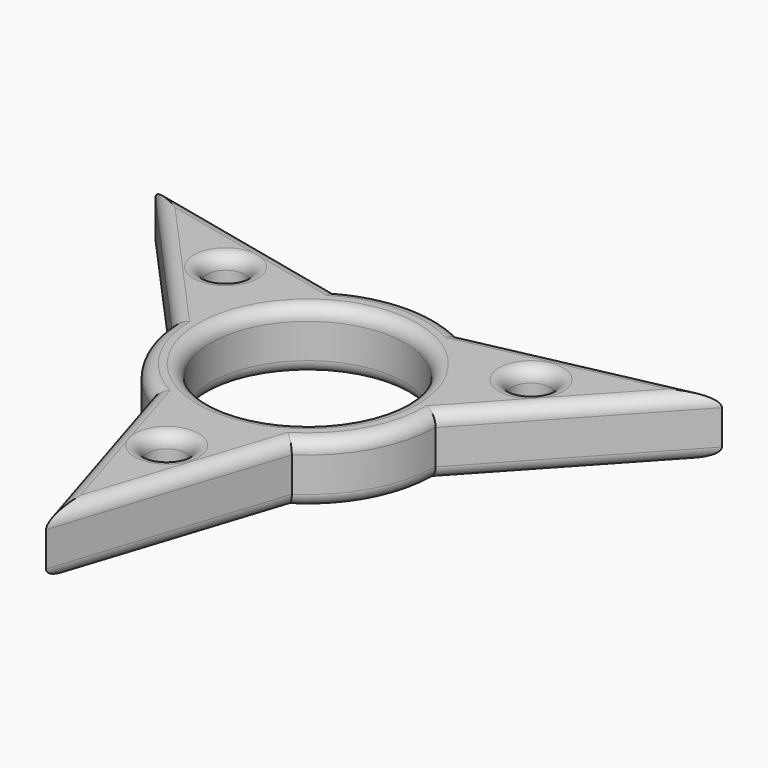
from build123d import *

# Parameters (mm, degrees)
F0_R          = 2.2
F0_R_2        = 11.2
F1_DEPTH      = 7
F2_T4_DEPTH   = 34.0623272755
F2_S5_R       = 15
F2_T6_DEPTH   = 19
F2_T10_ANGLE  = 84.4962693164
F2_T16_DEPTH  = 33.6377133372
F2_S17_R      = 15
F2_T18_DEPTH  = 19
F2_T22_DEPTH  = 34.0623272755
F2_S23_R      = 15
F2_T24_DEPTH  = 19
F2_T28_ANGLE  = 84.4962693164
F2_T34_DEPTH  = 33.6377133372
F2_S35_R      = 15
F2_T36_DEPTH  = 19
F2_T40_DEPTH  = 34.0623272755
F2_S41_R      = 15
F2_T42_DEPTH  = 19
F2_T46_ANGLE  = 84.4962693164
F2_T52_DEPTH  = 33.6377133372
F2_S53_R      = 15
F2_T54_DEPTH  = 19
F2_T66_DEPTH  = 34.0623272755
F2_S67_R      = 15
F2_T68_DEPTH  = 19
F2_T72_ANGLE  = 84.4962693164
F2_T78_DEPTH  = 33.6377133372
F2_S79_R      = 15
F2_T80_DEPTH  = 19
F2_T84_DEPTH  = 34.0623272755
F2_S85_R      = 15
F2_T86_DEPTH  = 19
F2_T90_ANGLE  = 84.4962693164
F2_T96_DEPTH  = 33.6377133372
F2_S97_R      = 15
F2_T98_DEPTH  = 19
F2_T102_DEPTH = 34.0623272755
F2_S103_R     = 15
F2_T104_DEPTH = 19
F2_T108_ANGLE = 84.4962693164
F2_T114_DEPTH = 33.6377133372
F2_S115_R     = 15
F2_T116_DEPTH = 19
F2_T129_DEPTH = 34.0623272755
F2_S130_R     = 15
F2_T131_DEPTH = 19
F2_T134_ANGLE = 84.4962693164
F2_T142_ANGLE = 84.4962693164
F2_T147_DEPTH = 33.6377133372
F2_S148_R     = 15
F2_T149_DEPTH = 19
F2_T155_DEPTH = 34.0623272755
F2_S156_R     = 15
F2_T157_DEPTH = 19
F2_T160_ANGLE = 84.4962693164
F2_T168_ANGLE = 84.4962693164
F2_T173_DEPTH = 33.6377133372
F2_S174_R     = 15
F2_T175_DEPTH = 19
F2_T181_DEPTH = 34.0623272755
F2_S182_R     = 15
F2_T183_DEPTH = 19
F2_T186_ANGLE = 84.4962693164
F2_T194_ANGLE = 84.4962693164
F2_T199_DEPTH = 33.6377133372
F2_S200_R     = 15
F2_T201_DEPTH = 19
F2_T207_DEPTH = 34.0623272755
F2_S208_R     = 15
F2_T209_DEPTH = 19
F2_T212_ANGLE = 84.4962693164
F2_T220_ANGLE = 84.4962693164
F2_T225_DEPTH = 33.6377133372
F2_S226_R     = 15
F2_T227_DEPTH = 19
F2_T233_DEPTH = 34.0623272755
F2_S234_R     = 15
F2_T235_DEPTH = 19
F2_T238_ANGLE = 84.4962693164
F2_T246_ANGLE = 84.4962693164
F2_T251_DEPTH = 33.6377133372
F2_S252_R     = 15
F2_T253_DEPTH = 19
F2_T259_DEPTH = 34.0623272755
F2_S260_R     = 15
F2_T261_DEPTH = 19
F2_T264_ANGLE = 84.4962693164
F2_T272_ANGLE = 84.4962693164
F2_T277_DEPTH = 33.6377133372
F2_S278_R     = 15
F2_T279_DEPTH = 19


# Not quite as in the source:
# - a fillet or chamfer that OpenCascade refuses, or shapes differently, is made with other operations: its cross-section is extruded or revolved along the edge and cut away or added


with BuildPart() as f1:
    # F0 (on Top) → F1 (new body)
    with BuildSketch(Plane.XY):
        with BuildLine():
            Line((-32.7569814166, 18.9122520387), (-14.9774534352, -0.8221244411))
            ThreePointArc((-14.9774534352, -0.8221244411), (-12.8488944768, -7.7398908729), (-7.7287556481, -12.8555955184))
            Line((-7.7287556481, -12.8555955184), (0, -37.8245040774))
            Line((0, -37.8245040774), (8.2007073687, -12.5597929383))
            ThreePointArc((8.2007073687, -12.5597929383), (13.1273893569, -7.2575235909), (14.9976501237, -0.2655009717))
            Line((14.9976501237, -0.2655009717), (32.7569814166, 18.9122520387))
            Line((32.7569814166, 18.9122520387), (6.7767460665, 13.3819173794))
            ThreePointArc((6.7767460665, 13.3819173794), (-0.2784948801, 14.9974144639), (-7.2688944757, 13.1210964901))
            Line((-7.2688944757, 13.1210964901), (-32.7569814166, 18.9122520387))
        make_face()
        with Locations((0, -20.3903708607)):
            Circle(F0_R, mode=Mode.SUBTRACT)
        Circle(F0_R_2, mode=Mode.SUBTRACT)
        with Locations((-17.6585791579, 10.1951854303)):
            Circle(F0_R, mode=Mode.SUBTRACT)
        with Locations((17.6585791579, 10.1951854303)):
            Circle(F0_R, mode=Mode.SUBTRACT)
    extrude(amount=F1_DEPTH)

    # F2: fillet of radius 1.5 on 26 edges, made by hand


with BuildPart() as f2_tool2:
    # F2_s3 → F2_t4 (new body)
    with BuildSketch(Plane(origin=(-26.5911251268, 29.5148034764, 0), x_dir=(0, 0, 1), z_dir=(0.6693512883, -0.7429460632, 0))):
        with BuildLine():
            ThreePointArc((5.5, 11.6777301208), (6.5606601718, 11.2383902926), (7, 10.1777301208))
            Line((7, 10.1777301208), (7, 11.6777301208))
            Line((7, 11.6777301208), (5.5, 11.6777301208))
        make_face()
    extrude(amount=F2_T4_DEPTH)

    # F2_s5 → F2_t6 (cut, symmetric)
    with BuildSketch(Plane.XY.offset(6.2)):
        Circle(F2_S5_R)
    extrude(amount=F2_T6_DEPTH, both=True, mode=Mode.SUBTRACT)


with BuildPart() as f1_1:
    add(f1.part)

    # F2_t1: cut F2_tool2
    add(f2_tool2.part, mode=Mode.SUBTRACT)


with BuildPart() as f2_tool8:
    # F2_s9 → F2_t10 (revolve)
    with BuildSketch(Plane(origin=(0, 0, 0), x_dir=(0, 0, 1), z_dir=(0.1939655707, 0.9810083371, 0))):
        with BuildLine():
            ThreePointArc((5.5, -15), (6.5606601718, -14.5606601718), (7, -13.5))
            Line((7, -13.5), (7, -15))
            Line((7, -15), (5.5, -15))
        make_face()
    revolve(axis=Axis((0, 0, 7), (0, 0, 1)), revolution_arc=F2_T10_ANGLE)

    split(bisect_by=Plane(origin=(-8.6759236209, -7.8165037005, 0), x_dir=(0, 0, 1), z_dir=(-0.7429460632, -0.6693512883, 0)), keep=Keep.TOP)

    split(bisect_by=Plane(origin=(-10.6843276365, -3.3071752965, 0), x_dir=(0, 0, 1), z_dir=(-0.9552828221, -0.2956936419, 0)), keep=Keep.TOP)


with BuildPart() as f1_2:
    add(f1_1.part)

    # F2_t7: cut F2_tool8
    add(f2_tool8.part, mode=Mode.SUBTRACT)


with BuildPart() as f2_tool14:
    # F2_s15 → F2_t16 (new body)
    with BuildSketch(Plane(origin=(1.8467208313, -5.9661096392, 0), x_dir=(0, 0, 1), z_dir=(0.2956936419, -0.9552828221, 0))):
        with BuildLine():
            ThreePointArc((5.5, 11.1844653644), (6.5606601718, 10.7451255361), (7, 9.6844653644))
            Line((7, 9.6844653644), (7, 11.1844653644))
            Line((7, 11.1844653644), (5.5, 11.1844653644))
        make_face()
    extrude(amount=F2_T16_DEPTH)

    # F2_s17 → F2_t18 (cut, symmetric)
    with BuildSketch(Plane.XY.offset(6.2)):
        Circle(F2_S17_R)
    extrude(amount=F2_T18_DEPTH, both=True, mode=Mode.SUBTRACT)


with BuildPart() as f1_3:
    add(f1_2.part)

    # F2_t13: cut F2_tool14
    add(f2_tool14.part, mode=Mode.SUBTRACT)


with BuildPart() as f2_tool20:
    # F2_s21 → F2_t22 (new body)
    with BuildSketch(Plane(origin=(-12.2650070349, -37.7859916132, 0), x_dir=(0, 0, 1), z_dir=(0.3087345203, 0.9511482513, 0))):
        with BuildLine():
            ThreePointArc((5.5, 11.6777301208), (6.5606601718, 11.2383902926), (7, 10.1777301208))
            Line((7, 10.1777301208), (7, 11.6777301208))
            Line((7, 11.6777301208), (5.5, 11.6777301208))
        make_face()
    extrude(amount=F2_T22_DEPTH)

    # F2_s23 → F2_t24 (cut, symmetric)
    with BuildSketch(Plane.XY.offset(6.2)):
        Circle(F2_S23_R)
    extrude(amount=F2_T24_DEPTH, both=True, mode=Mode.SUBTRACT)


with BuildPart() as f1_4:
    add(f1_3.part)

    # F2_t19: cut F2_tool20
    add(f2_tool20.part, mode=Mode.SUBTRACT)


with BuildPart() as f2_tool26:
    # F2_s27 → F2_t28 (revolve)
    with BuildSketch(Plane(origin=(0, 0, 0), x_dir=(0, 0, 1), z_dir=(-0.9465609266, -0.3225250569, 0))):
        with BuildLine():
            ThreePointArc((5.5, -15), (6.5606601718, -14.5606601718), (7, -13.5))
            Line((7, -13.5), (7, -15))
            Line((7, -15), (5.5, -15))
        make_face()
    revolve(axis=Axis((0, 0, 7), (0, 0, 1)), revolution_arc=F2_T28_ANGLE)

    split(bisect_by=Plane(origin=(11.1072525839, -3.6053184067, 0), x_dir=(0, 0, 1), z_dir=(0.9511482513, -0.3087345203, 0)), keep=Keep.TOP)

    split(bisect_by=Plane(origin=(8.2062616398, -7.5993115074, 0), x_dir=(0, 0, 1), z_dir=(0.7337196167, -0.6794523707, 0)), keep=Keep.TOP)


with BuildPart() as f1_5:
    add(f1_4.part)

    # F2_t25: cut F2_tool26
    add(f2_tool26.part, mode=Mode.SUBTRACT)


with BuildPart() as f2_tool32:
    # F2_s33 → F2_t34 (new body)
    with BuildSketch(Plane(origin=(4.2434420936, 4.5823619732, 0), x_dir=(0, 0, 1), z_dir=(0.6794523707, 0.7337196167, 0))):
        with BuildLine():
            ThreePointArc((5.5, 11.1844653644), (6.5606601718, 10.7451255361), (7, 9.6844653644))
            Line((7, 9.6844653644), (7, 11.1844653644))
            Line((7, 11.1844653644), (5.5, 11.1844653644))
        make_face()
    extrude(amount=F2_T34_DEPTH)

    # F2_s35 → F2_t36 (cut, symmetric)
    with BuildSketch(Plane.XY.offset(6.2)):
        Circle(F2_S35_R)
    extrude(amount=F2_T36_DEPTH, both=True, mode=Mode.SUBTRACT)


with BuildPart() as f1_6:
    add(f1_5.part)

    # F2_t31: cut F2_tool32
    add(f2_tool32.part, mode=Mode.SUBTRACT)


with BuildPart() as f2_tool38:
    # F2_s39 → F2_t40 (new body)
    with BuildSketch(Plane(origin=(38.8561321616, 8.2711881368, 0), x_dir=(0, 0, 1), z_dir=(-0.9780858085, -0.2082021881, 0))):
        with BuildLine():
            ThreePointArc((5.5, 11.6777301208), (6.5606601718, 11.2383902926), (7, 10.1777301208))
            Line((7, 10.1777301208), (7, 11.6777301208))
            Line((7, 11.6777301208), (5.5, 11.6777301208))
        make_face()
    extrude(amount=F2_T40_DEPTH)

    # F2_s41 → F2_t42 (cut, symmetric)
    with BuildSketch(Plane.XY.offset(6.2)):
        Circle(F2_S41_R)
    extrude(amount=F2_T42_DEPTH, both=True, mode=Mode.SUBTRACT)


with BuildPart() as f1_7:
    add(f1_6.part)

    # F2_t37: cut F2_tool38
    add(f2_tool38.part, mode=Mode.SUBTRACT)


with BuildPart() as f2_tool44:
    # F2_s45 → F2_t46 (revolve)
    with BuildSketch(Plane(origin=(0, 0, 0), x_dir=(0, 0, 1), z_dir=(0.7525953559, -0.6584832802, 0))):
        with BuildLine():
            ThreePointArc((5.5, -15), (6.5606601718, -14.5606601718), (7, -13.5))
            Line((7, -13.5), (7, -15))
            Line((7, -15), (5.5, -15))
        make_face()
    revolve(axis=Axis((0, 0, 7), (0, 0, 1)), revolution_arc=F2_T46_ANGLE)

    split(bisect_by=Plane(origin=(-2.431328963, 11.4218221072, 0), x_dir=(0, 0, 1), z_dir=(-0.2082021881, 0.9780858085, 0)), keep=Keep.TOP)

    split(bisect_by=Plane(origin=(2.4780659967, 10.9064868038, 0), x_dir=(0, 0, 1), z_dir=(0.2215632054, 0.9751460127, 0)), keep=Keep.TOP)


with BuildPart() as f1_8:
    add(f1_7.part)

    # F2_t43: cut F2_tool44
    add(f2_tool44.part, mode=Mode.SUBTRACT)


with BuildPart() as f2_tool50:
    # F2_s51 → F2_t52 (new body)
    with BuildSketch(Plane(origin=(-6.0901629249, 1.383747666, 0), x_dir=(0, 0, 1), z_dir=(-0.9751460127, 0.2215632054, 0))):
        with BuildLine():
            ThreePointArc((5.5, 11.1844653644), (6.5606601718, 10.7451255361), (7, 9.6844653644))
            Line((7, 9.6844653644), (7, 11.1844653644))
            Line((7, 11.1844653644), (5.5, 11.1844653644))
        make_face()
    extrude(amount=F2_T52_DEPTH)

    # F2_s53 → F2_t54 (cut, symmetric)
    with BuildSketch(Plane.XY.offset(6.2)):
        Circle(F2_S53_R)
    extrude(amount=F2_T54_DEPTH, both=True, mode=Mode.SUBTRACT)


with BuildPart() as f1_9:
    add(f1_8.part)

    # F2_t49: cut F2_tool50
    add(f2_tool50.part, mode=Mode.SUBTRACT)

    # F2_s55 → F2_t56 (revolve, cut)
    with BuildSketch(Plane.XZ.offset(20.3903708607)):
        with BuildLine():
            ThreePointArc((2.2, 5.5), (2.6393398282, 6.5606601718), (3.7, 7))
            Line((3.7, 7), (2.2, 7))
            Line((2.2, 7), (2.2, 5.5))
        make_face()
    revolve(axis=Axis((0, -20.3903708607, 7), (0, 0, 1)), mode=Mode.SUBTRACT)

    # F2_s57 → F2_t58 (revolve, cut)
    with BuildSketch(Plane.XZ):
        with BuildLine():
            ThreePointArc((11.2, 5.5), (11.6393398282, 6.5606601718), (12.7, 7))
            Line((12.7, 7), (11.2, 7))
            Line((11.2, 7), (11.2, 5.5))
        make_face()
    revolve(axis=Axis((0, 0, 7), (0, 0, 1)), mode=Mode.SUBTRACT)

    # F2_s59 → F2_t60 (revolve, cut)
    with BuildSketch(Plane.XZ.offset(-10.1951854303)):
        with BuildLine():
            ThreePointArc((-15.4585791579, 5.5), (-15.0192393297, 6.5606601718), (-13.9585791579, 7))
            Line((-13.9585791579, 7), (-15.4585791579, 7))
            Line((-15.4585791579, 7), (-15.4585791579, 5.5))
        make_face()
    revolve(axis=Axis((-17.6585791579, 10.1951854303, 7), (0, 0, 1)), mode=Mode.SUBTRACT)

    # F2_s61 → F2_t62 (revolve, cut)
    with BuildSketch(Plane.XZ.offset(-10.1951854303)):
        with BuildLine():
            ThreePointArc((19.8585791579, 5.5), (20.2979189862, 6.5606601718), (21.3585791579, 7))
            Line((21.3585791579, 7), (19.8585791579, 7))
            Line((19.8585791579, 7), (19.8585791579, 5.5))
        make_face()
    revolve(axis=Axis((17.6585791579, 10.1951854303, 7), (0, 0, 1)), mode=Mode.SUBTRACT)


with BuildPart() as f2_tool64:
    # F2_s65 → F2_t66 (new body)
    with BuildSketch(Plane(origin=(-26.5911251268, 29.5148034764, 0), x_dir=(0, 0, 1), z_dir=(0.6693512883, -0.7429460632, 0))):
        with BuildLine():
            ThreePointArc((1.5, 11.6777301208), (0.4393398282, 11.2383902926), (0, 10.1777301208))
            Line((0, 10.1777301208), (0, 11.6777301208))
            Line((0, 11.6777301208), (1.5, 11.6777301208))
        make_face()
    extrude(amount=F2_T66_DEPTH)

    # F2_s67 → F2_t68 (cut, symmetric)
    with BuildSketch(Plane.XY.offset(0.7)):
        Circle(F2_S67_R)
    extrude(amount=F2_T68_DEPTH, both=True, mode=Mode.SUBTRACT)


with BuildPart() as f1_10:
    add(f1_9.part)

    # F2_t63: cut F2_tool64
    add(f2_tool64.part, mode=Mode.SUBTRACT)


with BuildPart() as f2_tool70:
    # F2_s71 → F2_t72 (revolve)
    with BuildSketch(Plane(origin=(0, 0, 0), x_dir=(0, 0, 1), z_dir=(0.1939655707, 0.9810083371, 0))):
        with BuildLine():
            ThreePointArc((1.5, -15), (0.4393398282, -14.5606601718), (0, -13.5))
            Line((0, -13.5), (0, -15))
            Line((0, -15), (1.5, -15))
        make_face()
    revolve(axis=Axis((0, 0, 0), (0, 0, 1)), revolution_arc=F2_T72_ANGLE)

    split(bisect_by=Plane(origin=(-8.6759236209, -7.8165037005, 0), x_dir=(0, 0, 1), z_dir=(-0.7429460632, -0.6693512883, 0)), keep=Keep.TOP)

    split(bisect_by=Plane(origin=(-10.6843276365, -3.3071752965, 0), x_dir=(0, 0, 1), z_dir=(-0.9552828221, -0.2956936419, 0)), keep=Keep.TOP)


with BuildPart() as f1_11:
    add(f1_10.part)

    # F2_t69: cut F2_tool70
    add(f2_tool70.part, mode=Mode.SUBTRACT)


with BuildPart() as f2_tool76:
    # F2_s77 → F2_t78 (new body)
    with BuildSketch(Plane(origin=(1.8467208313, -5.9661096392, 0), x_dir=(0, 0, 1), z_dir=(0.2956936419, -0.9552828221, 0))):
        with BuildLine():
            ThreePointArc((1.5, 11.1844653644), (0.4393398282, 10.7451255361), (0, 9.6844653644))
            Line((0, 9.6844653644), (0, 11.1844653644))
            Line((0, 11.1844653644), (1.5, 11.1844653644))
        make_face()
    extrude(amount=F2_T78_DEPTH)

    # F2_s79 → F2_t80 (cut, symmetric)
    with BuildSketch(Plane.XY.offset(0.7)):
        Circle(F2_S79_R)
    extrude(amount=F2_T80_DEPTH, both=True, mode=Mode.SUBTRACT)


with BuildPart() as f1_12:
    add(f1_11.part)

    # F2_t75: cut F2_tool76
    add(f2_tool76.part, mode=Mode.SUBTRACT)


with BuildPart() as f2_tool82:
    # F2_s83 → F2_t84 (new body)
    with BuildSketch(Plane(origin=(-12.2650070349, -37.7859916132, 0), x_dir=(0, 0, 1), z_dir=(0.3087345203, 0.9511482513, 0))):
        with BuildLine():
            ThreePointArc((1.5, 11.6777301208), (0.4393398282, 11.2383902926), (0, 10.1777301208))
            Line((0, 10.1777301208), (0, 11.6777301208))
            Line((0, 11.6777301208), (1.5, 11.6777301208))
        make_face()
    extrude(amount=F2_T84_DEPTH)

    # F2_s85 → F2_t86 (cut, symmetric)
    with BuildSketch(Plane.XY.offset(0.7)):
        Circle(F2_S85_R)
    extrude(amount=F2_T86_DEPTH, both=True, mode=Mode.SUBTRACT)


with BuildPart() as f1_13:
    add(f1_12.part)

    # F2_t81: cut F2_tool82
    add(f2_tool82.part, mode=Mode.SUBTRACT)


with BuildPart() as f2_tool88:
    # F2_s89 → F2_t90 (revolve)
    with BuildSketch(Plane(origin=(0, 0, 0), x_dir=(0, 0, 1), z_dir=(-0.9465609266, -0.3225250569, 0))):
        with BuildLine():
            ThreePointArc((1.5, -15), (0.4393398282, -14.5606601718), (0, -13.5))
            Line((0, -13.5), (0, -15))
            Line((0, -15), (1.5, -15))
        make_face()
    revolve(axis=Axis((0, 0, 0), (0, 0, 1)), revolution_arc=F2_T90_ANGLE)

    split(bisect_by=Plane(origin=(11.1072525839, -3.6053184067, 0), x_dir=(0, 0, 1), z_dir=(0.9511482513, -0.3087345203, 0)), keep=Keep.TOP)

    split(bisect_by=Plane(origin=(8.2062616398, -7.5993115074, 0), x_dir=(0, 0, 1), z_dir=(0.7337196167, -0.6794523707, 0)), keep=Keep.TOP)


with BuildPart() as f1_14:
    add(f1_13.part)

    # F2_t87: cut F2_tool88
    add(f2_tool88.part, mode=Mode.SUBTRACT)


with BuildPart() as f2_tool94:
    # F2_s95 → F2_t96 (new body)
    with BuildSketch(Plane(origin=(4.2434420936, 4.5823619732, 0), x_dir=(0, 0, 1), z_dir=(0.6794523707, 0.7337196167, 0))):
        with BuildLine():
            ThreePointArc((1.5, 11.1844653644), (0.4393398282, 10.7451255361), (0, 9.6844653644))
            Line((0, 9.6844653644), (0, 11.1844653644))
            Line((0, 11.1844653644), (1.5, 11.1844653644))
        make_face()
    extrude(amount=F2_T96_DEPTH)

    # F2_s97 → F2_t98 (cut, symmetric)
    with BuildSketch(Plane.XY.offset(0.7)):
        Circle(F2_S97_R)
    extrude(amount=F2_T98_DEPTH, both=True, mode=Mode.SUBTRACT)


with BuildPart() as f1_15:
    add(f1_14.part)

    # F2_t93: cut F2_tool94
    add(f2_tool94.part, mode=Mode.SUBTRACT)


with BuildPart() as f2_tool100:
    # F2_s101 → F2_t102 (new body)
    with BuildSketch(Plane(origin=(38.8561321616, 8.2711881368, 0), x_dir=(0, 0, 1), z_dir=(-0.9780858085, -0.2082021881, 0))):
        with BuildLine():
            ThreePointArc((1.5, 11.6777301208), (0.4393398282, 11.2383902926), (0, 10.1777301208))
            Line((0, 10.1777301208), (0, 11.6777301208))
            Line((0, 11.6777301208), (1.5, 11.6777301208))
        make_face()
    extrude(amount=F2_T102_DEPTH)

    # F2_s103 → F2_t104 (cut, symmetric)
    with BuildSketch(Plane.XY.offset(0.7)):
        Circle(F2_S103_R)
    extrude(amount=F2_T104_DEPTH, both=True, mode=Mode.SUBTRACT)


with BuildPart() as f1_16:
    add(f1_15.part)

    # F2_t99: cut F2_tool100
    add(f2_tool100.part, mode=Mode.SUBTRACT)


with BuildPart() as f2_tool106:
    # F2_s107 → F2_t108 (revolve)
    with BuildSketch(Plane(origin=(0, 0, 0), x_dir=(0, 0, 1), z_dir=(0.7525953559, -0.6584832802, 0))):
        with BuildLine():
            ThreePointArc((1.5, -15), (0.4393398282, -14.5606601718), (0, -13.5))
            Line((0, -13.5), (0, -15))
            Line((0, -15), (1.5, -15))
        make_face()
    revolve(axis=Axis((0, 0, 0), (0, 0, 1)), revolution_arc=F2_T108_ANGLE)

    split(bisect_by=Plane(origin=(-2.431328963, 11.4218221072, 0), x_dir=(0, 0, 1), z_dir=(-0.2082021881, 0.9780858085, 0)), keep=Keep.TOP)

    split(bisect_by=Plane(origin=(2.4780659967, 10.9064868038, 0), x_dir=(0, 0, 1), z_dir=(0.2215632054, 0.9751460127, 0)), keep=Keep.TOP)


with BuildPart() as f1_17:
    add(f1_16.part)

    # F2_t105: cut F2_tool106
    add(f2_tool106.part, mode=Mode.SUBTRACT)


with BuildPart() as f2_tool112:
    # F2_s113 → F2_t114 (new body)
    with BuildSketch(Plane(origin=(-6.0901629249, 1.383747666, 0), x_dir=(0, 0, 1), z_dir=(-0.9751460127, 0.2215632054, 0))):
        with BuildLine():
            ThreePointArc((1.5, 11.1844653644), (0.4393398282, 10.7451255361), (0, 9.6844653644))
            Line((0, 9.6844653644), (0, 11.1844653644))
            Line((0, 11.1844653644), (1.5, 11.1844653644))
        make_face()
    extrude(amount=F2_T114_DEPTH)

    # F2_s115 → F2_t116 (cut, symmetric)
    with BuildSketch(Plane.XY.offset(0.7)):
        Circle(F2_S115_R)
    extrude(amount=F2_T116_DEPTH, both=True, mode=Mode.SUBTRACT)


with BuildPart() as f1_18:
    add(f1_17.part)

    # F2_t111: cut F2_tool112
    add(f2_tool112.part, mode=Mode.SUBTRACT)

    # F2_s117 → F2_t118 (revolve, cut)
    with BuildSketch(Plane.XZ.offset(20.3903708607)):
        with BuildLine():
            ThreePointArc((2.2, 1.5), (2.6393398282, 0.4393398282), (3.7, 0))
            Line((3.7, 0), (2.2, 0))
            Line((2.2, 0), (2.2, 1.5))
        make_face()
    revolve(axis=Axis((0, -20.3903708607, 0), (0, 0, 1)), mode=Mode.SUBTRACT)

    # F2_s119 → F2_t120 (revolve, cut)
    with BuildSketch(Plane.XZ):
        with BuildLine():
            ThreePointArc((11.2, 1.5), (11.6393398282, 0.4393398282), (12.7, 0))
            Line((12.7, 0), (11.2, 0))
            Line((11.2, 0), (11.2, 1.5))
        make_face()
    revolve(axis=Axis((0, 0, 0), (0, 0, 1)), mode=Mode.SUBTRACT)

    # F2_s121 → F2_t122 (revolve, cut)
    with BuildSketch(Plane.XZ.offset(-10.1951854303)):
        with BuildLine():
            ThreePointArc((-15.4585791579, 1.5), (-15.0192393297, 0.4393398282), (-13.9585791579, 0))
            Line((-13.9585791579, 0), (-15.4585791579, 0))
            Line((-15.4585791579, 0), (-15.4585791579, 1.5))
        make_face()
    revolve(axis=Axis((-17.6585791579, 10.1951854303, 0), (0, 0, 1)), mode=Mode.SUBTRACT)

    # F2_s123 → F2_t124 (revolve, cut)
    with BuildSketch(Plane.XZ.offset(-10.1951854303)):
        with BuildLine():
            ThreePointArc((19.8585791579, 1.5), (20.2979189862, 0.4393398282), (21.3585791579, 0))
            Line((21.3585791579, 0), (19.8585791579, 0))
            Line((19.8585791579, 0), (19.8585791579, 1.5))
        make_face()
    revolve(axis=Axis((17.6585791579, 10.1951854303, 0), (0, 0, 1)), mode=Mode.SUBTRACT)


with BuildPart() as f2_tool127:
    # F2_s128 → F2_t129 (new body)
    with BuildSketch(Plane(origin=(-26.5911251268, 29.5148034764, 0), x_dir=(0, 0, 1), z_dir=(0.6693512883, -0.7429460632, 0))):
        with BuildLine():
            ThreePointArc((5.5, 11.6777301208), (6.5606601718, 11.2383902926), (7, 10.1777301208))
            Line((7, 10.1777301208), (7, 11.6777301208))
            Line((7, 11.6777301208), (5.5, 11.6777301208))
        make_face()
    extrude(amount=F2_T129_DEPTH)

    # F2_s130 → F2_t131 (intersect, symmetric)
    with BuildSketch(Plane.XY.offset(6.2)):
        Circle(F2_S130_R)
    extrude(amount=F2_T131_DEPTH, both=True, mode=Mode.INTERSECT)


with BuildPart() as f2_tool132:
    # F2_s133 → F2_t134 (revolve)
    with BuildSketch(Plane(origin=(0, 0, 0), x_dir=(0, 0, 1), z_dir=(0.1939655707, 0.9810083371, 0))):
        with BuildLine():
            ThreePointArc((5.5, -15), (6.5606601718, -14.5606601718), (7, -13.5))
            Line((7, -13.5), (7, -15))
            Line((7, -15), (5.5, -15))
        make_face()
    revolve(axis=Axis((0, 0, 7), (0, 0, 1)), revolution_arc=F2_T134_ANGLE)

    split(bisect_by=Plane(origin=(-8.6759236209, -7.8165037005, 0), x_dir=(0, 0, 1), z_dir=(0.7429460632, 0.6693512883, 0)), keep=Keep.TOP)

    split(bisect_by=Plane(origin=(-10.6843276365, -3.3071752965, 0), x_dir=(0, 0, 1), z_dir=(-0.9552828221, -0.2956936419, 0)), keep=Keep.TOP)


with BuildPart() as f2_tool127_1:
    add(f2_tool127.part)

    # F2_t137: intersect F2_tool132
    add(f2_tool132.part, mode=Mode.INTERSECT)


with BuildPart() as f1_19:
    add(f1_18.part)

    # F2_t125: cut F2_tool127
    add(f2_tool127_1.part, mode=Mode.SUBTRACT)


with BuildPart() as f2_tool140:
    # F2_s141 → F2_t142 (revolve)
    with BuildSketch(Plane(origin=(0, 0, 0), x_dir=(0, 0, 1), z_dir=(0.1939655707, 0.9810083371, 0))):
        with BuildLine():
            ThreePointArc((5.5, -15), (6.5606601718, -14.5606601718), (7, -13.5))
            Line((7, -13.5), (7, -15))
            Line((7, -15), (5.5, -15))
        make_face()
    revolve(axis=Axis((0, 0, 7), (0, 0, 1)), revolution_arc=F2_T142_ANGLE)

    split(bisect_by=Plane(origin=(-8.6759236209, -7.8165037005, 0), x_dir=(0, 0, 1), z_dir=(-0.7429460632, -0.6693512883, 0)), keep=Keep.TOP)

    split(bisect_by=Plane(origin=(-10.6843276365, -3.3071752965, 0), x_dir=(0, 0, 1), z_dir=(0.9552828221, 0.2956936419, 0)), keep=Keep.TOP)


with BuildPart() as f2_tool145:
    # F2_s146 → F2_t147 (new body)
    with BuildSketch(Plane(origin=(1.8467208313, -5.9661096392, 0), x_dir=(0, 0, 1), z_dir=(0.2956936419, -0.9552828221, 0))):
        with BuildLine():
            ThreePointArc((5.5, 11.1844653644), (6.5606601718, 10.7451255361), (7, 9.6844653644))
            Line((7, 9.6844653644), (7, 11.1844653644))
            Line((7, 11.1844653644), (5.5, 11.1844653644))
        make_face()
    extrude(amount=F2_T147_DEPTH)

    # F2_s148 → F2_t149 (intersect, symmetric)
    with BuildSketch(Plane.XY.offset(6.2)):
        Circle(F2_S148_R)
    extrude(amount=F2_T149_DEPTH, both=True, mode=Mode.INTERSECT)


with BuildPart() as f2_tool140_1:
    add(f2_tool140.part)

    # F2_t150: intersect F2_tool145
    add(f2_tool145.part, mode=Mode.INTERSECT)


with BuildPart() as f1_20:
    add(f1_19.part)

    # F2_t138: cut F2_tool140
    add(f2_tool140_1.part, mode=Mode.SUBTRACT)


with BuildPart() as f2_tool153:
    # F2_s154 → F2_t155 (new body)
    with BuildSketch(Plane(origin=(-12.2650070349, -37.7859916132, 0), x_dir=(0, 0, 1), z_dir=(0.3087345203, 0.9511482513, 0))):
        with BuildLine():
            ThreePointArc((5.5, 11.6777301208), (6.5606601718, 11.2383902926), (7, 10.1777301208))
            Line((7, 10.1777301208), (7, 11.6777301208))
            Line((7, 11.6777301208), (5.5, 11.6777301208))
        make_face()
    extrude(amount=F2_T155_DEPTH)

    # F2_s156 → F2_t157 (intersect, symmetric)
    with BuildSketch(Plane.XY.offset(6.2)):
        Circle(F2_S156_R)
    extrude(amount=F2_T157_DEPTH, both=True, mode=Mode.INTERSECT)


with BuildPart() as f2_tool158:
    # F2_s159 → F2_t160 (revolve)
    with BuildSketch(Plane(origin=(0, 0, 0), x_dir=(0, 0, 1), z_dir=(-0.9465609266, -0.3225250569, 0))):
        with BuildLine():
            ThreePointArc((5.5, -15), (6.5606601718, -14.5606601718), (7, -13.5))
            Line((7, -13.5), (7, -15))
            Line((7, -15), (5.5, -15))
        make_face()
    revolve(axis=Axis((0, 0, 7), (0, 0, 1)), revolution_arc=F2_T160_ANGLE)

    split(bisect_by=Plane(origin=(11.1072525839, -3.6053184067, 0), x_dir=(0, 0, 1), z_dir=(-0.9511482513, 0.3087345203, 0)), keep=Keep.TOP)

    split(bisect_by=Plane(origin=(8.2062616398, -7.5993115074, 0), x_dir=(0, 0, 1), z_dir=(0.7337196167, -0.6794523707, 0)), keep=Keep.TOP)


with BuildPart() as f2_tool153_1:
    add(f2_tool153.part)

    # F2_t163: intersect F2_tool158
    add(f2_tool158.part, mode=Mode.INTERSECT)


with BuildPart() as f1_21:
    add(f1_20.part)

    # F2_t151: cut F2_tool153
    add(f2_tool153_1.part, mode=Mode.SUBTRACT)


with BuildPart() as f2_tool166:
    # F2_s167 → F2_t168 (revolve)
    with BuildSketch(Plane(origin=(0, 0, 0), x_dir=(0, 0, 1), z_dir=(-0.9465609266, -0.3225250569, 0))):
        with BuildLine():
            ThreePointArc((5.5, -15), (6.5606601718, -14.5606601718), (7, -13.5))
            Line((7, -13.5), (7, -15))
            Line((7, -15), (5.5, -15))
        make_face()
    revolve(axis=Axis((0, 0, 7), (0, 0, 1)), revolution_arc=F2_T168_ANGLE)

    split(bisect_by=Plane(origin=(11.1072525839, -3.6053184067, 0), x_dir=(0, 0, 1), z_dir=(0.9511482513, -0.3087345203, 0)), keep=Keep.TOP)

    split(bisect_by=Plane(origin=(8.2062616398, -7.5993115074, 0), x_dir=(0, 0, 1), z_dir=(-0.7337196167, 0.6794523707, 0)), keep=Keep.TOP)


with BuildPart() as f2_tool171:
    # F2_s172 → F2_t173 (new body)
    with BuildSketch(Plane(origin=(4.2434420936, 4.5823619732, 0), x_dir=(0, 0, 1), z_dir=(0.6794523707, 0.7337196167, 0))):
        with BuildLine():
            ThreePointArc((5.5, 11.1844653644), (6.5606601718, 10.7451255361), (7, 9.6844653644))
            Line((7, 9.6844653644), (7, 11.1844653644))
            Line((7, 11.1844653644), (5.5, 11.1844653644))
        make_face()
    extrude(amount=F2_T173_DEPTH)

    # F2_s174 → F2_t175 (intersect, symmetric)
    with BuildSketch(Plane.XY.offset(6.2)):
        Circle(F2_S174_R)
    extrude(amount=F2_T175_DEPTH, both=True, mode=Mode.INTERSECT)


with BuildPart() as f2_tool166_1:
    add(f2_tool166.part)

    # F2_t176: intersect F2_tool171
    add(f2_tool171.part, mode=Mode.INTERSECT)


with BuildPart() as f1_22:
    add(f1_21.part)

    # F2_t164: cut F2_tool166
    add(f2_tool166_1.part, mode=Mode.SUBTRACT)


with BuildPart() as f2_tool179:
    # F2_s180 → F2_t181 (new body)
    with BuildSketch(Plane(origin=(38.8561321616, 8.2711881368, 0), x_dir=(0, 0, 1), z_dir=(-0.9780858085, -0.2082021881, 0))):
        with BuildLine():
            ThreePointArc((5.5, 11.6777301208), (6.5606601718, 11.2383902926), (7, 10.1777301208))
            Line((7, 10.1777301208), (7, 11.6777301208))
            Line((7, 11.6777301208), (5.5, 11.6777301208))
        make_face()
    extrude(amount=F2_T181_DEPTH)

    # F2_s182 → F2_t183 (intersect, symmetric)
    with BuildSketch(Plane.XY.offset(6.2)):
        Circle(F2_S182_R)
    extrude(amount=F2_T183_DEPTH, both=True, mode=Mode.INTERSECT)


with BuildPart() as f2_tool184:
    # F2_s185 → F2_t186 (revolve)
    with BuildSketch(Plane(origin=(0, 0, 0), x_dir=(0, 0, 1), z_dir=(0.7525953559, -0.6584832802, 0))):
        with BuildLine():
            ThreePointArc((5.5, -15), (6.5606601718, -14.5606601718), (7, -13.5))
            Line((7, -13.5), (7, -15))
            Line((7, -15), (5.5, -15))
        make_face()
    revolve(axis=Axis((0, 0, 7), (0, 0, 1)), revolution_arc=F2_T186_ANGLE)

    split(bisect_by=Plane(origin=(-2.431328963, 11.4218221072, 0), x_dir=(0, 0, 1), z_dir=(0.2082021881, -0.9780858085, 0)), keep=Keep.TOP)

    split(bisect_by=Plane(origin=(2.4780659967, 10.9064868038, 0), x_dir=(0, 0, 1), z_dir=(0.2215632054, 0.9751460127, 0)), keep=Keep.TOP)


with BuildPart() as f2_tool179_1:
    add(f2_tool179.part)

    # F2_t189: intersect F2_tool184
    add(f2_tool184.part, mode=Mode.INTERSECT)


with BuildPart() as f1_23:
    add(f1_22.part)

    # F2_t177: cut F2_tool179
    add(f2_tool179_1.part, mode=Mode.SUBTRACT)


with BuildPart() as f2_tool192:
    # F2_s193 → F2_t194 (revolve)
    with BuildSketch(Plane(origin=(0, 0, 0), x_dir=(0, 0, 1), z_dir=(0.7525953559, -0.6584832802, 0))):
        with BuildLine():
            ThreePointArc((5.5, -15), (6.5606601718, -14.5606601718), (7, -13.5))
            Line((7, -13.5), (7, -15))
            Line((7, -15), (5.5, -15))
        make_face()
    revolve(axis=Axis((0, 0, 7), (0, 0, 1)), revolution_arc=F2_T194_ANGLE)

    split(bisect_by=Plane(origin=(-2.431328963, 11.4218221072, 0), x_dir=(0, 0, 1), z_dir=(-0.2082021881, 0.9780858085, 0)), keep=Keep.TOP)

    split(bisect_by=Plane(origin=(2.4780659967, 10.9064868038, 0), x_dir=(0, 0, 1), z_dir=(-0.2215632054, -0.9751460127, 0)), keep=Keep.TOP)


with BuildPart() as f2_tool197:
    # F2_s198 → F2_t199 (new body)
    with BuildSketch(Plane(origin=(-6.0901629249, 1.383747666, 0), x_dir=(0, 0, 1), z_dir=(-0.9751460127, 0.2215632054, 0))):
        with BuildLine():
            ThreePointArc((5.5, 11.1844653644), (6.5606601718, 10.7451255361), (7, 9.6844653644))
            Line((7, 9.6844653644), (7, 11.1844653644))
            Line((7, 11.1844653644), (5.5, 11.1844653644))
        make_face()
    extrude(amount=F2_T199_DEPTH)

    # F2_s200 → F2_t201 (intersect, symmetric)
    with BuildSketch(Plane.XY.offset(6.2)):
        Circle(F2_S200_R)
    extrude(amount=F2_T201_DEPTH, both=True, mode=Mode.INTERSECT)


with BuildPart() as f2_tool192_1:
    add(f2_tool192.part)

    # F2_t202: intersect F2_tool197
    add(f2_tool197.part, mode=Mode.INTERSECT)


with BuildPart() as f1_24:
    add(f1_23.part)

    # F2_t190: cut F2_tool192
    add(f2_tool192_1.part, mode=Mode.SUBTRACT)


with BuildPart() as f2_tool205:
    # F2_s206 → F2_t207 (new body)
    with BuildSketch(Plane(origin=(-26.5911251268, 29.5148034764, 0), x_dir=(0, 0, 1), z_dir=(0.6693512883, -0.7429460632, 0))):
        with BuildLine():
            ThreePointArc((1.5, 11.6777301208), (0.4393398282, 11.2383902926), (0, 10.1777301208))
            Line((0, 10.1777301208), (0, 11.6777301208))
            Line((0, 11.6777301208), (1.5, 11.6777301208))
        make_face()
    extrude(amount=F2_T207_DEPTH)

    # F2_s208 → F2_t209 (intersect, symmetric)
    with BuildSketch(Plane.XY.offset(0.7)):
        Circle(F2_S208_R)
    extrude(amount=F2_T209_DEPTH, both=True, mode=Mode.INTERSECT)


with BuildPart() as f2_tool210:
    # F2_s211 → F2_t212 (revolve)
    with BuildSketch(Plane(origin=(0, 0, 0), x_dir=(0, 0, 1), z_dir=(0.1939655707, 0.9810083371, 0))):
        with BuildLine():
            ThreePointArc((1.5, -15), (0.4393398282, -14.5606601718), (0, -13.5))
            Line((0, -13.5), (0, -15))
            Line((0, -15), (1.5, -15))
        make_face()
    revolve(axis=Axis((0, 0, 0), (0, 0, 1)), revolution_arc=F2_T212_ANGLE)

    split(bisect_by=Plane(origin=(-8.6759236209, -7.8165037005, 0), x_dir=(0, 0, 1), z_dir=(0.7429460632, 0.6693512883, 0)), keep=Keep.TOP)

    split(bisect_by=Plane(origin=(-10.6843276365, -3.3071752965, 0), x_dir=(0, 0, 1), z_dir=(-0.9552828221, -0.2956936419, 0)), keep=Keep.TOP)


with BuildPart() as f2_tool205_1:
    add(f2_tool205.part)

    # F2_t215: intersect F2_tool210
    add(f2_tool210.part, mode=Mode.INTERSECT)


with BuildPart() as f1_25:
    add(f1_24.part)

    # F2_t203: cut F2_tool205
    add(f2_tool205_1.part, mode=Mode.SUBTRACT)


with BuildPart() as f2_tool218:
    # F2_s219 → F2_t220 (revolve)
    with BuildSketch(Plane(origin=(0, 0, 0), x_dir=(0, 0, 1), z_dir=(0.1939655707, 0.9810083371, 0))):
        with BuildLine():
            ThreePointArc((1.5, -15), (0.4393398282, -14.5606601718), (0, -13.5))
            Line((0, -13.5), (0, -15))
            Line((0, -15), (1.5, -15))
        make_face()
    revolve(axis=Axis((0, 0, 0), (0, 0, 1)), revolution_arc=F2_T220_ANGLE)

    split(bisect_by=Plane(origin=(-8.6759236209, -7.8165037005, 0), x_dir=(0, 0, 1), z_dir=(-0.7429460632, -0.6693512883, 0)), keep=Keep.TOP)

    split(bisect_by=Plane(origin=(-10.6843276365, -3.3071752965, 0), x_dir=(0, 0, 1), z_dir=(0.9552828221, 0.2956936419, 0)), keep=Keep.TOP)


with BuildPart() as f2_tool223:
    # F2_s224 → F2_t225 (new body)
    with BuildSketch(Plane(origin=(1.8467208313, -5.9661096392, 0), x_dir=(0, 0, 1), z_dir=(0.2956936419, -0.9552828221, 0))):
        with BuildLine():
            ThreePointArc((1.5, 11.1844653644), (0.4393398282, 10.7451255361), (0, 9.6844653644))
            Line((0, 9.6844653644), (0, 11.1844653644))
            Line((0, 11.1844653644), (1.5, 11.1844653644))
        make_face()
    extrude(amount=F2_T225_DEPTH)

    # F2_s226 → F2_t227 (intersect, symmetric)
    with BuildSketch(Plane.XY.offset(0.7)):
        Circle(F2_S226_R)
    extrude(amount=F2_T227_DEPTH, both=True, mode=Mode.INTERSECT)


with BuildPart() as f2_tool218_1:
    add(f2_tool218.part)

    # F2_t228: intersect F2_tool223
    add(f2_tool223.part, mode=Mode.INTERSECT)


with BuildPart() as f1_26:
    add(f1_25.part)

    # F2_t216: cut F2_tool218
    add(f2_tool218_1.part, mode=Mode.SUBTRACT)


with BuildPart() as f2_tool231:
    # F2_s232 → F2_t233 (new body)
    with BuildSketch(Plane(origin=(-12.2650070349, -37.7859916132, 0), x_dir=(0, 0, 1), z_dir=(0.3087345203, 0.9511482513, 0))):
        with BuildLine():
            ThreePointArc((1.5, 11.6777301208), (0.4393398282, 11.2383902926), (0, 10.1777301208))
            Line((0, 10.1777301208), (0, 11.6777301208))
            Line((0, 11.6777301208), (1.5, 11.6777301208))
        make_face()
    extrude(amount=F2_T233_DEPTH)

    # F2_s234 → F2_t235 (intersect, symmetric)
    with BuildSketch(Plane.XY.offset(0.7)):
        Circle(F2_S234_R)
    extrude(amount=F2_T235_DEPTH, both=True, mode=Mode.INTERSECT)


with BuildPart() as f2_tool236:
    # F2_s237 → F2_t238 (revolve)
    with BuildSketch(Plane(origin=(0, 0, 0), x_dir=(0, 0, 1), z_dir=(-0.9465609266, -0.3225250569, 0))):
        with BuildLine():
            ThreePointArc((1.5, -15), (0.4393398282, -14.5606601718), (0, -13.5))
            Line((0, -13.5), (0, -15))
            Line((0, -15), (1.5, -15))
        make_face()
    revolve(axis=Axis((0, 0, 0), (0, 0, 1)), revolution_arc=F2_T238_ANGLE)

    split(bisect_by=Plane(origin=(11.1072525839, -3.6053184067, 0), x_dir=(0, 0, 1), z_dir=(-0.9511482513, 0.3087345203, 0)), keep=Keep.TOP)

    split(bisect_by=Plane(origin=(8.2062616398, -7.5993115074, 0), x_dir=(0, 0, 1), z_dir=(0.7337196167, -0.6794523707, 0)), keep=Keep.TOP)


with BuildPart() as f2_tool231_1:
    add(f2_tool231.part)

    # F2_t241: intersect F2_tool236
    add(f2_tool236.part, mode=Mode.INTERSECT)


with BuildPart() as f1_27:
    add(f1_26.part)

    # F2_t229: cut F2_tool231
    add(f2_tool231_1.part, mode=Mode.SUBTRACT)


with BuildPart() as f2_tool244:
    # F2_s245 → F2_t246 (revolve)
    with BuildSketch(Plane(origin=(0, 0, 0), x_dir=(0, 0, 1), z_dir=(-0.9465609266, -0.3225250569, 0))):
        with BuildLine():
            ThreePointArc((1.5, -15), (0.4393398282, -14.5606601718), (0, -13.5))
            Line((0, -13.5), (0, -15))
            Line((0, -15), (1.5, -15))
        make_face()
    revolve(axis=Axis((0, 0, 0), (0, 0, 1)), revolution_arc=F2_T246_ANGLE)

    split(bisect_by=Plane(origin=(11.1072525839, -3.6053184067, 0), x_dir=(0, 0, 1), z_dir=(0.9511482513, -0.3087345203, 0)), keep=Keep.TOP)

    split(bisect_by=Plane(origin=(8.2062616398, -7.5993115074, 0), x_dir=(0, 0, 1), z_dir=(-0.7337196167, 0.6794523707, 0)), keep=Keep.TOP)


with BuildPart() as f2_tool249:
    # F2_s250 → F2_t251 (new body)
    with BuildSketch(Plane(origin=(4.2434420936, 4.5823619732, 0), x_dir=(0, 0, 1), z_dir=(0.6794523707, 0.7337196167, 0))):
        with BuildLine():
            ThreePointArc((1.5, 11.1844653644), (0.4393398282, 10.7451255361), (0, 9.6844653644))
            Line((0, 9.6844653644), (0, 11.1844653644))
            Line((0, 11.1844653644), (1.5, 11.1844653644))
        make_face()
    extrude(amount=F2_T251_DEPTH)

    # F2_s252 → F2_t253 (intersect, symmetric)
    with BuildSketch(Plane.XY.offset(0.7)):
        Circle(F2_S252_R)
    extrude(amount=F2_T253_DEPTH, both=True, mode=Mode.INTERSECT)


with BuildPart() as f2_tool244_1:
    add(f2_tool244.part)

    # F2_t254: intersect F2_tool249
    add(f2_tool249.part, mode=Mode.INTERSECT)


with BuildPart() as f1_28:
    add(f1_27.part)

    # F2_t242: cut F2_tool244
    add(f2_tool244_1.part, mode=Mode.SUBTRACT)


with BuildPart() as f2_tool257:
    # F2_s258 → F2_t259 (new body)
    with BuildSketch(Plane(origin=(38.8561321616, 8.2711881368, 0), x_dir=(0, 0, 1), z_dir=(-0.9780858085, -0.2082021881, 0))):
        with BuildLine():
            ThreePointArc((1.5, 11.6777301208), (0.4393398282, 11.2383902926), (0, 10.1777301208))
            Line((0, 10.1777301208), (0, 11.6777301208))
            Line((0, 11.6777301208), (1.5, 11.6777301208))
        make_face()
    extrude(amount=F2_T259_DEPTH)

    # F2_s260 → F2_t261 (intersect, symmetric)
    with BuildSketch(Plane.XY.offset(0.7)):
        Circle(F2_S260_R)
    extrude(amount=F2_T261_DEPTH, both=True, mode=Mode.INTERSECT)


with BuildPart() as f2_tool262:
    # F2_s263 → F2_t264 (revolve)
    with BuildSketch(Plane(origin=(0, 0, 0), x_dir=(0, 0, 1), z_dir=(0.7525953559, -0.6584832802, 0))):
        with BuildLine():
            ThreePointArc((1.5, -15), (0.4393398282, -14.5606601718), (0, -13.5))
            Line((0, -13.5), (0, -15))
            Line((0, -15), (1.5, -15))
        make_face()
    revolve(axis=Axis((0, 0, 0), (0, 0, 1)), revolution_arc=F2_T264_ANGLE)

    split(bisect_by=Plane(origin=(-2.431328963, 11.4218221072, 0), x_dir=(0, 0, 1), z_dir=(0.2082021881, -0.9780858085, 0)), keep=Keep.TOP)

    split(bisect_by=Plane(origin=(2.4780659967, 10.9064868038, 0), x_dir=(0, 0, 1), z_dir=(0.2215632054, 0.9751460127, 0)), keep=Keep.TOP)


with BuildPart() as f2_tool257_1:
    add(f2_tool257.part)

    # F2_t267: intersect F2_tool262
    add(f2_tool262.part, mode=Mode.INTERSECT)


with BuildPart() as f1_29:
    add(f1_28.part)

    # F2_t255: cut F2_tool257
    add(f2_tool257_1.part, mode=Mode.SUBTRACT)


with BuildPart() as f2_tool270:
    # F2_s271 → F2_t272 (revolve)
    with BuildSketch(Plane(origin=(0, 0, 0), x_dir=(0, 0, 1), z_dir=(0.7525953559, -0.6584832802, 0))):
        with BuildLine():
            ThreePointArc((1.5, -15), (0.4393398282, -14.5606601718), (0, -13.5))
            Line((0, -13.5), (0, -15))
            Line((0, -15), (1.5, -15))
        make_face()
    revolve(axis=Axis((0, 0, 0), (0, 0, 1)), revolution_arc=F2_T272_ANGLE)

    split(bisect_by=Plane(origin=(-2.431328963, 11.4218221072, 0), x_dir=(0, 0, 1), z_dir=(-0.2082021881, 0.9780858085, 0)), keep=Keep.TOP)

    split(bisect_by=Plane(origin=(2.4780659967, 10.9064868038, 0), x_dir=(0, 0, 1), z_dir=(-0.2215632054, -0.9751460127, 0)), keep=Keep.TOP)


with BuildPart() as f2_tool275:
    # F2_s276 → F2_t277 (new body)
    with BuildSketch(Plane(origin=(-6.0901629249, 1.383747666, 0), x_dir=(0, 0, 1), z_dir=(-0.9751460127, 0.2215632054, 0))):
        with BuildLine():
            ThreePointArc((1.5, 11.1844653644), (0.4393398282, 10.7451255361), (0, 9.6844653644))
            Line((0, 9.6844653644), (0, 11.1844653644))
            Line((0, 11.1844653644), (1.5, 11.1844653644))
        make_face()
    extrude(amount=F2_T277_DEPTH)

    # F2_s278 → F2_t279 (intersect, symmetric)
    with BuildSketch(Plane.XY.offset(0.7)):
        Circle(F2_S278_R)
    extrude(amount=F2_T279_DEPTH, both=True, mode=Mode.INTERSECT)


with BuildPart() as f2_tool270_1:
    add(f2_tool270.part)

    # F2_t280: intersect F2_tool275
    add(f2_tool275.part, mode=Mode.INTERSECT)


with BuildPart() as f1_30:
    add(f1_29.part)

    # F2_t268: cut F2_tool270
    add(f2_tool270_1.part, mode=Mode.SUBTRACT)


solid = f1_30.part
